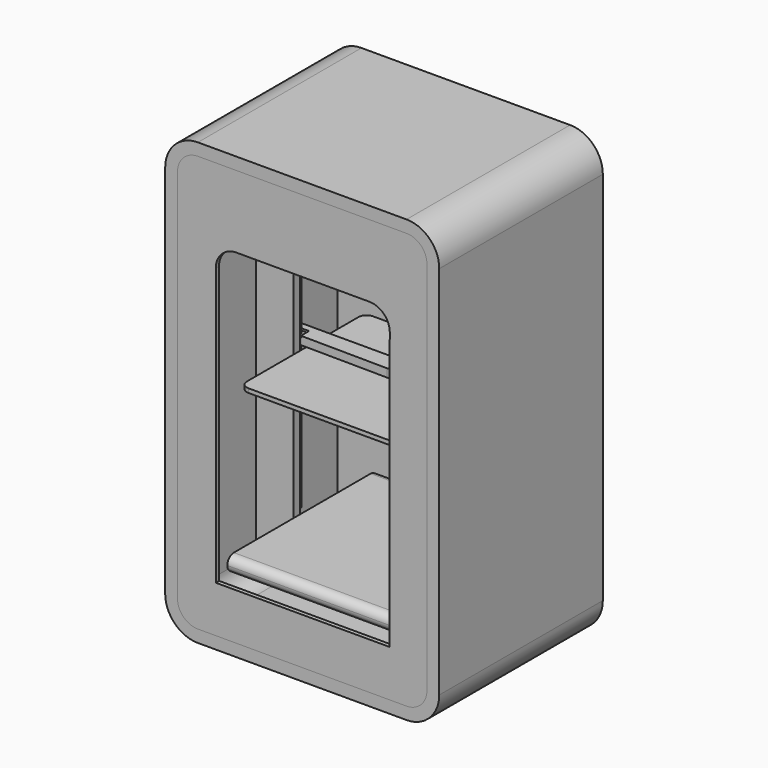
from build123d import *

# Parameters (mm, degrees)
F1_DEPTH    = 1
F2_DEPTH    = 25
F4_DEPTH    = 1
F6_DEPTH    = 1
F8_DEPTH    = 20
F9_T1_DEPTH = 50
F10_W       = 4.2359828949
F10_H       = 1.5884938184
F11_DEPTH   = 35
F12_W       = 39.7970937192
F12_H       = 38.108728826
F13_DEPTH   = 1
F14_R       = 2
F16_DEPTH   = 2
F17_DEPTH   = 1.5


# Not quite as in the source:
# - a fillet or chamfer that OpenCascade refuses, or shapes differently, is made with other operations: its cross-section is extruded or revolved along the edge and cut away or added


with BuildPart() as f1:
    # F0 (on Front) → F1 (new body, symmetric)
    with BuildSketch(Plane.XZ):
        with BuildLine():
            Line((-25.5111035705, -50.8920401335), (25.5111035705, -50.8920401335))
            ThreePointArc((25.5111035705, -50.8920401335), (29.0466374764, -49.4275740394), (30.5111035705, -45.8920401335))
            Line((30.5111035705, -45.8920401335), (30.5111035705, 45.8920401335))
            ThreePointArc((30.5111035705, 45.8920401335), (29.0466374764, 49.4275740394), (25.5111035705, 50.8920401335))
            Line((25.5111035705, 50.8920401335), (-25.5111035705, 50.8920401335))
            ThreePointArc((-25.5111035705, 50.8920401335), (-29.0466374764, 49.4275740394), (-30.5111035705, 45.8920401335))
            Line((-30.5111035705, 45.8920401335), (-30.5111035705, -45.8920401335))
            ThreePointArc((-30.5111035705, -45.8920401335), (-29.0466374764, -49.4275740394), (-25.5111035705, -50.8920401335))
        make_face()
        with BuildLine():
            Line((-16.3457122445, 39.7970937192), (16.3457122445, 39.7970937192))
            ThreePointArc((16.3457122445, 39.7970937192), (19.8812461504, 38.3326276252), (21.3457122445, 34.7970937192))
            Line((21.3457122445, 34.7970937192), (21.3457122445, -39.7970937192))
            Line((21.3457122445, -39.7970937192), (-21.3457122445, -39.7970937192))
            Line((-21.3457122445, -39.7970937192), (-21.3457122445, 34.7970937192))
            ThreePointArc((-21.3457122445, 34.7970937192), (-19.8812461504, 38.3326276252), (-16.3457122445, 39.7970937192))
        make_face(mode=Mode.SUBTRACT)
    extrude(amount=F1_DEPTH, both=True)


with BuildPart() as f2:
    # F0 (on Front) → F2 (new body, symmetric)
    with BuildSketch(Plane.XZ):
        with BuildLine():
            Line((33.5111035705, -45.8920401335), (33.5111035705, 45.8920401335))
            ThreePointArc((33.5111035705, 45.8920401335), (31.16795782, 51.548894383), (25.5111035705, 53.8920401335))
            Line((25.5111035705, 53.8920401335), (-25.5111035705, 53.8920401335))
            ThreePointArc((-25.5111035705, 53.8920401335), (-31.16795782, 51.548894383), (-33.5111035705, 45.8920401335))
            Line((-33.5111035705, 45.8920401335), (-33.5111035705, -45.8920401335))
            ThreePointArc((-33.5111035705, -45.8920401335), (-31.16795782, -51.548894383), (-25.5111035705, -53.8920401335))
            Line((-25.5111035705, -53.8920401335), (25.5111035705, -53.8920401335))
            ThreePointArc((25.5111035705, -53.8920401335), (31.16795782, -51.548894383), (33.5111035705, -45.8920401335))
        make_face()
        with BuildLine():
            ThreePointArc((30.5111035705, -45.8920401335), (29.0466374764, -49.4275740394), (25.5111035705, -50.8920401335))
            Line((25.5111035705, -50.8920401335), (-25.5111035705, -50.8920401335))
            ThreePointArc((-25.5111035705, -50.8920401335), (-29.0466374764, -49.4275740394), (-30.5111035705, -45.8920401335))
            Line((-30.5111035705, -45.8920401335), (-30.5111035705, 45.8920401335))
            ThreePointArc((-30.5111035705, 45.8920401335), (-29.0466374764, 49.4275740394), (-25.5111035705, 50.8920401335))
            Line((-25.5111035705, 50.8920401335), (25.5111035705, 50.8920401335))
            ThreePointArc((25.5111035705, 50.8920401335), (29.0466374764, 49.4275740394), (30.5111035705, 45.8920401335))
            Line((30.5111035705, 45.8920401335), (30.5111035705, -45.8920401335))
        make_face(mode=Mode.SUBTRACT)
    extrude(amount=F2_DEPTH, both=True)


with BuildPart() as f4:
    # F3 (on face) → F4 (new body)
    with BuildSketch(Plane.XZ.offset(25)):
        with BuildLine():
            ThreePointArc((30.5111035705, 45.8920401335), (29.0466374764, 49.4275740394), (25.5111035705, 50.8920401335))
            Line((25.5111035705, 50.8920401335), (-25.5111035705, 50.8920401335))
            ThreePointArc((-25.5111035705, 50.8920401335), (-29.0466374764, 49.4275740394), (-30.5111035705, 45.8920401335))
            Line((-30.5111035705, 45.8920401335), (-30.5111035705, -45.8920401335))
            ThreePointArc((-30.5111035705, -45.8920401335), (-29.0466374764, -49.4275740394), (-25.5111035705, -50.8920401335))
            Line((-25.5111035705, -50.8920401335), (25.5111035705, -50.8920401335))
            ThreePointArc((25.5111035705, -50.8920401335), (29.0466374764, -49.4275740394), (30.5111035705, -45.8920401335))
            Line((30.5111035705, -45.8920401335), (30.5111035705, 45.8920401335))
        make_face()
        with BuildLine():
            Line((21.4197138017, 28.1762804146), (21.3457085192, 19.8430334032))
            Line((21.3457085192, 19.8430334032), (21.3457085192, -39.5023338497))
            Line((21.3457085192, -39.5023338497), (-21.1417768151, -39.5023338497))
            Line((-21.1417768151, -39.5023338497), (-21.1417768151, 19.8430334032))
            Line((-21.1417768151, 19.8430334032), (-21.1417768151, 28.2206822932))
            ThreePointArc((-21.1417768151, 28.2206822932), (-19.677310721, 31.7562161991), (-16.1417768151, 33.2206822932))
            Line((-16.1417768151, 33.2206822932), (16.4199109583, 33.2206822932))
            ThreePointArc((16.4199109583, 33.2206822932), (19.9711086009, 31.7404827568), (21.4197138017, 28.1762804146))
        make_face(mode=Mode.SUBTRACT)
    extrude(amount=-F4_DEPTH)


with BuildPart() as f6:
    # F5 (on face) → F6 (new body)
    with BuildSketch(Plane(origin=(0, 25, 0), x_dir=(-1, 0, 0), z_dir=(0, 1, 0))):
        with BuildLine():
            ThreePointArc((30.5111035705, 45.8920401335), (29.0466374764, 49.4275740394), (25.5111035705, 50.8920401335))
            Line((25.5111035705, 50.8920401335), (-25.5111035705, 50.8920401335))
            ThreePointArc((-25.5111035705, 50.8920401335), (-29.0466374764, 49.4275740394), (-30.5111035705, 45.8920401335))
            Line((-30.5111035705, 45.8920401335), (-30.5111035705, -45.8920401335))
            ThreePointArc((-30.5111035705, -45.8920401335), (-29.0466374764, -49.4275740394), (-25.5111035705, -50.8920401335))
            Line((-25.5111035705, -50.8920401335), (25.5111035705, -50.8920401335))
            ThreePointArc((25.5111035705, -50.8920401335), (29.0466374764, -49.4275740394), (30.5111035705, -45.8920401335))
            Line((30.5111035705, -45.8920401335), (30.5111035705, 45.8920401335))
        make_face()
    extrude(amount=-F6_DEPTH)


with BuildPart() as f8:
    # F7 (on Right) → F8 (new body, symmetric)
    with BuildSketch(Plane.YZ):
        Polygon((-22.9129418731, -38.1699390709), (0, -38.1699390709), (22.9129418731, -38.1699390709), (22.9129418731, -34.3046039343), (0, -34.3046039343), (-22.9129418731, -34.3046039343), align=None)
    extrude(amount=F8_DEPTH, both=True)

    # F9: fillet of radius 2 on 4 edges, made by hand

    # F9_s2 → F9_t1 (cut)
    with BuildSketch(Plane.YZ.offset(-25)):
        with BuildLine():
            ThreePointArc((-22.9129418731, -36.3046039343), (-22.3271554354, -34.8903903719), (-20.9129418731, -34.3046039343))
            Line((-20.9129418731, -34.3046039343), (-22.9129418731, -34.3046039343))
            Line((-22.9129418731, -34.3046039343), (-22.9129418731, -36.3046039343))
        make_face()
        with BuildLine():
            ThreePointArc((-20.9129418731, -38.1699390709), (-22.3271554354, -37.5841526333), (-22.9129418731, -36.1699390709))
            Line((-22.9129418731, -36.1699390709), (-22.9129418731, -38.1699390709))
            Line((-22.9129418731, -38.1699390709), (-20.9129418731, -38.1699390709))
        make_face()
        with BuildLine():
            ThreePointArc((20.9129418731, -34.3046039343), (22.3271554354, -34.8903903719), (22.9129418731, -36.3046039343))
            Line((22.9129418731, -36.3046039343), (22.9129418731, -34.3046039343))
            Line((22.9129418731, -34.3046039343), (20.9129418731, -34.3046039343))
        make_face()
        with BuildLine():
            ThreePointArc((20.9129418731, -38.1699390709), (22.3271554354, -37.5841526333), (22.9129418731, -36.1699390709))
            Line((22.9129418731, -36.1699390709), (22.9129418731, -38.1699390709))
            Line((22.9129418731, -38.1699390709), (20.9129418731, -38.1699390709))
        make_face()
    extrude(amount=F9_T1_DEPTH, mode=Mode.SUBTRACT)


with BuildPart() as f11:
    # F10 (on Top) → F11 (new body, symmetric)
    with BuildSketch(Plane.XY):
        with Locations((24.545153603, 1.9773821114)):
            Rectangle(F10_W, F10_H)
    extrude(amount=F11_DEPTH, both=True)


with BuildPart() as f11b:
    # F10 (on Top) → F11, piece 2 (new body, symmetric)
    with BuildSketch(Plane.XY):
        with Locations((-24.545153603, 1.9773821114)):
            Rectangle(F10_W, F10_H)
    extrude(amount=F11_DEPTH, both=True)


with BuildPart() as f13:
    # F12 (on Top) → F13 (new body)
    with BuildSketch(Plane.XY):
        Rectangle(F12_W, F12_H)
    extrude(amount=F13_DEPTH)

    # F14
    f14_edges = [f13.edges().sort_by_distance(p)[0] for p in [
        (19.898547, -19.054364, 0.5),
        (-19.898547, -19.054364, 0.5),
        (-19.898547, 19.054364, 0.5),
        (19.898547, 19.054364, 0.5),
    ]]
    fillet(f14_edges, radius=F14_R)

    # F15 (on face) → F16 (join)
    with BuildSketch(Plane.XY.offset(1)):
        Polygon((19.8985468596, 5.3184535354), (19.8985468596, 1.1494957364), (21.2562642992, 1.1638099095), (21.2562642992, 3.6611582618), (27.9961694032, 3.6611582618), (27.9961694032, 5.3184535354), align=None)
        Polygon((0, 5.3184535354), (0, 0.9397089016), (19.8985468596, 1.1494957364), (19.8985468596, 5.3184535354), align=None)
        Polygon((-19.8985468596, 5.3184535354), (-19.8985468596, 1.1494957364), (0, 0.9397089016), (0, 5.3184535354), align=None)
        Polygon((-21.2562642992, 3.6611582618), (-21.2562642992, 1.1638099095), (-19.8985468596, 1.1494957364), (-19.8985468596, 5.3184535354), (-27.9961694032, 5.3184535354), (-27.9961694032, 3.6611582618), align=None)
    extrude(amount=F16_DEPTH)

    # F15 (on face) → F17 (join, symmetric)
    with BuildSketch(Plane.XY.offset(1)):
        Polygon((-22.4111061543, 2.8803967871), (-22.4111061543, 1.1638099095), (-21.2562642992, 1.1638099095), (-21.2562642992, 3.6611582618), (-27.9961694032, 3.6611582618), (-27.9961694032, 1.2822989374), (-26.8449559808, 1.2822989374), (-26.8449559808, 2.8803967871), align=None)
        Polygon((21.2562642992, 3.6611582618), (21.2562642992, 1.1638099095), (22.4111061543, 1.1638099095), (22.4111061543, 2.8803967871), (26.8449559808, 2.8803967871), (26.8449559808, 1.2822989374), (27.9961694032, 1.2822989374), (27.9961694032, 3.6611582618), align=None)
    extrude(amount=F17_DEPTH, both=True)


solid = Compound([f1.part, f2.part, f4.part, f6.part, f8.part, f11.part, f11b.part, f13.part])
